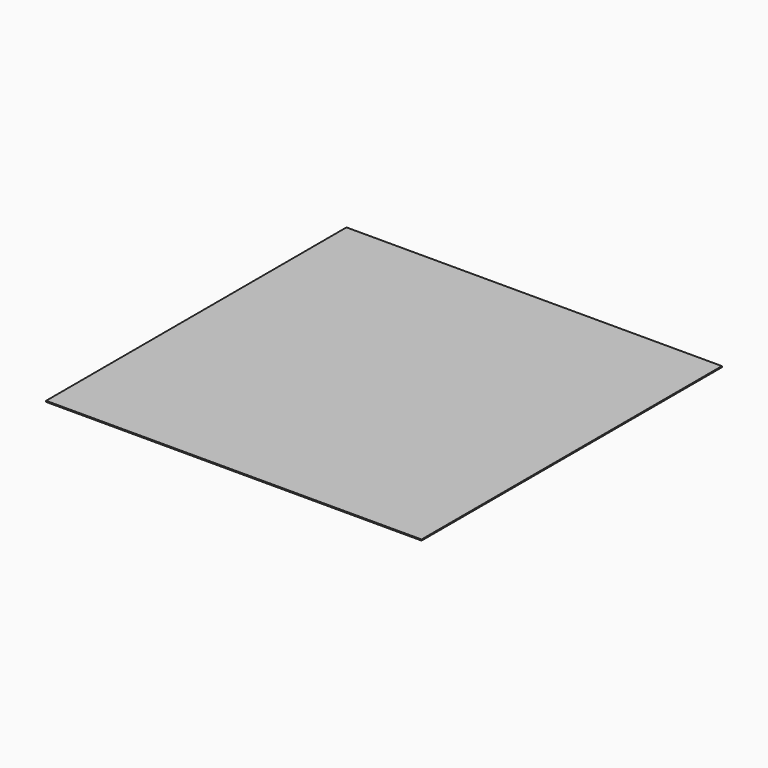
from build123d import *

# Parameters (mm, degrees)
F0_W     = 571.5
F0_H     = 571.5
F1_DEPTH = 1.5875


# Not quite as in the source:
# - a length typed as a fraction of an inch, garbled in the dataset ("3 / 203.2 mm" for 3/8 in), is restored


with BuildPart() as f1:
    # F0 (on Top) → F1 (new body)
    with BuildSketch(Plane.XY):
        with Locations((-181.3765061041, -6.8569388241)):
            Rectangle(F0_W, F0_H)
    extrude(amount=F1_DEPTH)


solid = f1.part
